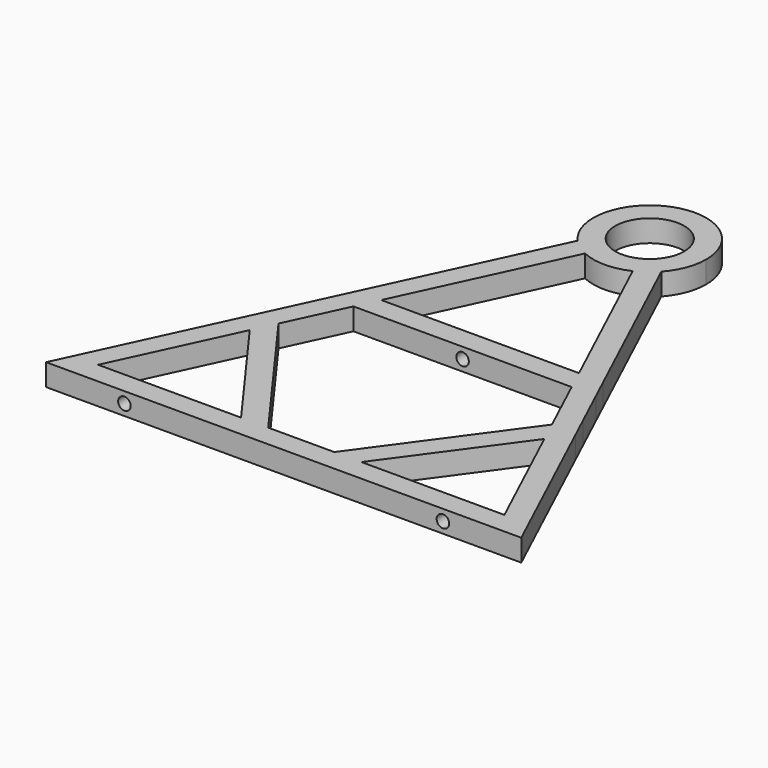
from build123d import *

# Parameters (mm, degrees)
F1_DEPTH = 7
F2_R     = 2
F3_DEPTH = 8
F4_R     = 2
F5_DEPTH = 8


# Not quite as in the source:
# - a feature names something its author has since deleted; it is built from what else it names


with BuildPart() as f1:
    # F0 (on Top) → F1 (new body)
    with BuildSketch(Plane.XY):
        with BuildLine():
            ThreePointArc((9.930189374, -4.7319487525), (7.7456068538, -7.8106065364), (4.6488008791, -9.9693856574))
            Line((4.6488008791, -9.9693856574), (7.6071287113, -16.3135401667))
            ThreePointArc((7.6071287113, -16.3135401667), (10.6923318533, -14.4801256741), (13.352485528, -12.0710865387))
            Line((13.352485528, -12.0710865387), (9.930189374, -4.7319487525))
        make_face()
        with BuildLine():
            Line((7.6071287113, -16.3135401667), (4.6488008791, -9.9693856574))
            ThreePointArc((4.6488008791, -9.9693856574), (0, -11), (-4.6488008791, -9.9693856574))
            Line((-4.6488008791, -9.9693856574), (-7.6071287113, -16.3135401667))
            ThreePointArc((-7.6071287113, -16.3135401667), (0, -18), (7.6071287113, -16.3135401667))
        make_face()
        with BuildLine():
            Line((-7.6071287113, -16.3135401667), (-4.6488008791, -9.9693856574))
            ThreePointArc((-4.6488008791, -9.9693856574), (-7.7456068538, -7.8106065364), (-9.930189374, -4.7319487525))
            Line((-9.930189374, -4.7319487525), (-13.352485528, -12.0710865387))
            ThreePointArc((-13.352485528, -12.0710865387), (-10.6923318533, -14.4801256741), (-7.6071287113, -16.3135401667))
        make_face()
        with BuildLine():
            ThreePointArc((13.352485528, -12.0710865387), (10.6923318533, -14.4801256741), (7.6071287113, -16.3135401667))
            Line((7.6071287113, -16.3135401667), (31.5509050579, -67.6611342449))
            Line((31.5509050579, -67.6611342449), (39.2745504906, -67.6611342449))
            Line((39.2745504906, -67.6611342449), (13.352485528, -12.0710865387))
        make_face()
        with BuildLine():
            ThreePointArc((11, 0), (10.7292143961, -2.4256872104), (9.930189374, -4.7319487525))
            Line((9.930189374, -4.7319487525), (13.352485528, -12.0710865387))
            ThreePointArc((13.352485528, -12.0710865387), (16.7979870744, -6.4674284107), (18, 0))
            ThreePointArc((18, 0), (-6.4674284107, 16.7979870744), (-13.352485528, -12.0710865387))
            Line((-13.352485528, -12.0710865387), (-9.930189374, -4.7319487525))
            ThreePointArc((-9.930189374, -4.7319487525), (-2.4256872104, 10.7292143961), (11, 0))
        make_face()
        with BuildLine():
            Line((-31.5509050579, -67.6611342449), (-7.6071287113, -16.3135401667))
            ThreePointArc((-7.6071287113, -16.3135401667), (-10.6923318533, -14.4801256741), (-13.352485528, -12.0710865387))
            Line((-13.352485528, -12.0710865387), (-39.2745504906, -67.6611342449))
            Line((-39.2745504906, -67.6611342449), (-31.5509050579, -67.6611342449))
        make_face()
        Polygon((39.2745504906, -67.6611342449), (31.5509050579, -67.6611342449), (34.8150586649, -74.6611342449), (42.5387040977, -74.6611342449), align=None)
        Polygon((34.8150586649, -74.6611342449), (31.5509050579, -67.6611342449), (-31.5509050579, -67.6611342449), (-34.8150586649, -74.6611342449), align=None)
        Polygon((-34.8150586649, -74.6611342449), (-31.5509050579, -67.6611342449), (-39.2745504906, -67.6611342449), (-42.5387040977, -74.6611342449), align=None)
        Polygon((42.5387040977, -74.6611342449), (34.8150586649, -74.6611342449), (43.6188979632, -93.5410285471), (48.3261309802, -87.0723112465), align=None)
        Polygon((-43.6188979632, -93.5410285471), (-34.8150586649, -74.6611342449), (-42.5387040977, -74.6611342449), (-48.3261309802, -87.0723112465), align=None)
        Polygon((48.3261309802, -87.0723112465), (43.6188979632, -93.5410285471), (46.9999060281, -100.7916237405), (51.7071390451, -94.3229064398), align=None)
        Polygon((46.9999060281, -100.7916237405), (43.6188979632, -93.5410285471), (10.5389814088, -138.9997147322), (19.1961886798, -138.9997147322), align=None)
        Polygon((-10.5389814088, -138.9997147322), (-43.6188979632, -93.5410285471), (-46.9999060281, -100.7916237405), (-19.1961886798, -138.9997147322), align=None)
        Polygon((-46.9999060281, -100.7916237405), (-43.6188979632, -93.5410285471), (-48.3261309802, -87.0723112465), (-51.7071390451, -94.3229064398), align=None)
        Polygon((51.7071390451, -94.3229064398), (46.9999060281, -100.7916237405), (64.816631461, -138.9997147322), (19.1961886798, -138.9997147322), (14.1023455596, -145.9997147322), (75.8044305008, -145.9997147322), align=None)
        Polygon((19.1961886798, -138.9997147322), (10.5389814088, -138.9997147322), (5.4451382885, -145.9997147322), (14.1023455596, -145.9997147322), align=None)
        Polygon((5.4451382885, -145.9997147322), (10.5389814088, -138.9997147322), (-10.5389814088, -138.9997147322), (-5.4451382885, -145.9997147322), align=None)
        Polygon((-64.816631461, -138.9997147322), (-46.9999060281, -100.7916237405), (-51.7071390451, -94.3229064398), (-75.8044305008, -145.9997147322), (-14.1023455596, -145.9997147322), (-19.1961886798, -138.9997147322), align=None)
        Polygon((-5.4451382885, -145.9997147322), (-10.5389814088, -138.9997147322), (-19.1961886798, -138.9997147322), (-14.1023455596, -145.9997147322), align=None)
    extrude(amount=F1_DEPTH)

    # F2 (on face) → F3 (cut)
    with BuildSketch(Plane(origin=(0, -67.6611342449, 0), x_dir=(-1, 0, 0), z_dir=(0, 1, 0))):
        with Locations((0, 3.5)):
            Circle(F2_R)
    extrude(amount=-F3_DEPTH, mode=Mode.SUBTRACT)

    # F4 (on face) → F5 (cut)
    with BuildSketch(Plane.XZ.offset(145.9997147322)):
        with Locations((-50.8044305008, 3.5)):
            Circle(F4_R)
        with Locations((50.8044305008, 3.5)):
            Circle(F4_R)
    extrude(amount=-F5_DEPTH, mode=Mode.SUBTRACT)


solid = f1.part
